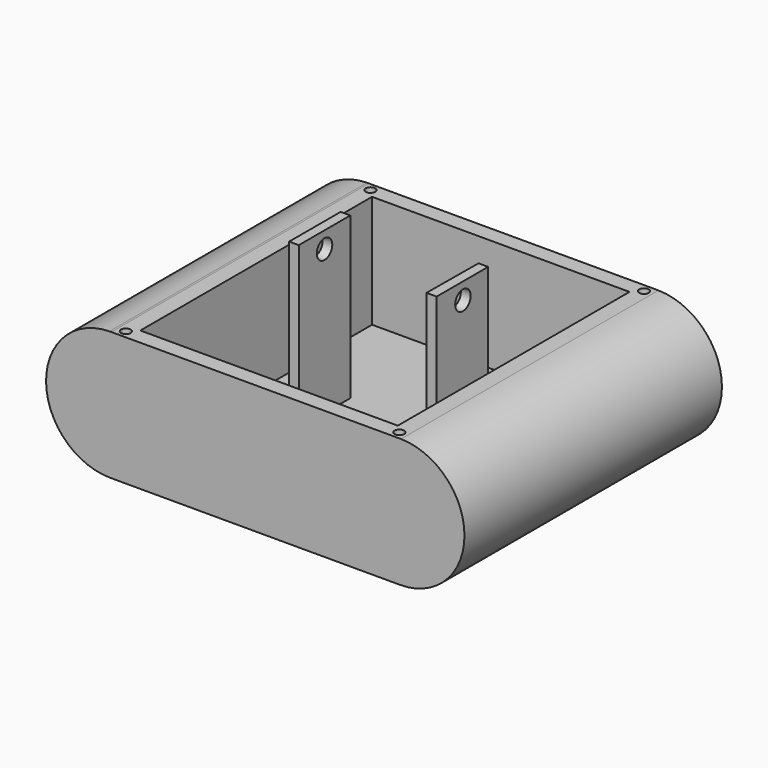
from build123d import *

# Parameters (mm, degrees)
F1_DEPTH = 50
F2_W     = 80
F2_H     = 90
F2_W_2   = 3
F2_H_2   = 20
F3_DEPTH = 35
F4_D     = 3
F4_DEPTH = 20
F4_TIP   = 0.9012909285
F5_R     = 5
F6_DEPTH = 10
F7_DEPTH = 15
F8_R     = 3
F9_DEPTH = 60


# Not quite as in the source:
# - a feature names something its author has since deleted; it is built from what else it names


with BuildPart() as f1:
    # F0 (on Front) → F1 (new body, symmetric)
    with BuildSketch(Plane.XZ):
        with BuildLine():
            Line((-59.7125668165, 19.9979344475), (-60.2874331835, 19.9979344475))
            ThreePointArc((-60.2874331835, 19.9979344475), (-79.9994836052, -0.1437203026), (-60, -20))
            ThreePointArc((-60, -20), (-45.8578643763, -14.1421356237), (-40, 0))
            ThreePointArc((-40, 0), (-45.756603922, 14.0401448769), (-59.7125668165, 19.9979344475))
        make_face()
        with BuildLine():
            ThreePointArc((-59.7125668165, 19.9979344475), (-60, 20), (-60.2874331835, 19.9979344475))
            Line((-60.2874331835, 19.9979344475), (-59.7125668165, 19.9979344475))
        make_face()
        with BuildLine():
            ThreePointArc((-40, 0), (-45.8578643763, -14.1421356237), (-60, -20))
            Line((-60, -20), (30, -20))
            ThreePointArc((30, -20), (10.0005163948, -0.1437203026), (29.7125668165, 19.9979344475))
            Line((29.7125668165, 19.9979344475), (-59.7125668165, 19.9979344475))
            ThreePointArc((-59.7125668165, 19.9979344475), (-45.756603922, 14.0401448769), (-40, 0))
        make_face()
        with BuildLine():
            ThreePointArc((29.7125668165, 19.9979344475), (10.0005163948, -0.1437203026), (30, -20))
            ThreePointArc((30, -20), (44.1421356237, -14.1421356237), (50, 0))
            ThreePointArc((50, 0), (44.243396078, 14.0401448769), (30.2874331835, 19.9979344475))
            Line((30.2874331835, 19.9979344475), (29.7125668165, 19.9979344475))
        make_face()
    extrude(amount=F1_DEPTH, both=True)

    # F2 (on face) → F3 (cut)
    with BuildSketch(Plane.XY.offset(19.9979344475)):
        with Locations((-14.7125668165, 0)):
            Rectangle(F2_W, F2_H)
        with Locations((-36.2125668165, 1.5482969955)):
            Rectangle(F2_W_2, F2_H_2, mode=Mode.SUBTRACT)
        Polygon((8.2874331835, 11.3340624973), (8.2874331835, -8.6665749961), (5.1278462474, -8.641347646), (5.2875288045, 11.3580148809), align=None, mode=Mode.SUBTRACT)
    extrude(amount=-F3_DEPTH, mode=Mode.SUBTRACT)

    # F4
    with Locations(Plane.XY.offset(19.9979344475)):
        with Locations((-57.2125668165, 47.5), (27.7874331835, 47.5), (27.7874331835, -47.5), (-57.2125668165, -47.5)):
            Hole(F4_D / 2, depth=F4_DEPTH)
            with Locations((0, 0, -(F4_DEPTH + F4_TIP / 2))):  # 118° drill point
                Cone(0, F4_D / 2, F4_TIP, mode=Mode.SUBTRACT)

    # F5 (on face) → F6 (cut)
    with BuildSketch(Plane(origin=(0, 50, 0), x_dir=(-1, 0, 0), z_dir=(0, 1, 0))):
        with Locations((-12.6515543088, 0)):
            Circle(F5_R)
    extrude(amount=-F6_DEPTH, mode=Mode.SUBTRACT)

    # F7 (add): faces of the model
    f7_faces = [f1.faces().sort_by_distance(p)[0] for p in [
        (-36.2125668165, 1.5482969955, 19.9979344475),
        (6.7472153787, 1.2596232378, 19.9979344475),
    ]]
    extrude(f7_faces, amount=F7_DEPTH)

    # F8 (on face) → F9 (cut)
    with BuildSketch(Plane(origin=(-37.7125668165, 0, 0), x_dir=(0, -1, 0), z_dir=(-1, 0, 0))):
        with Locations((-1.5482969955, 29.857664355)):
            Circle(F8_R)
    extrude(amount=-F9_DEPTH, mode=Mode.SUBTRACT)


solid = f1.part
